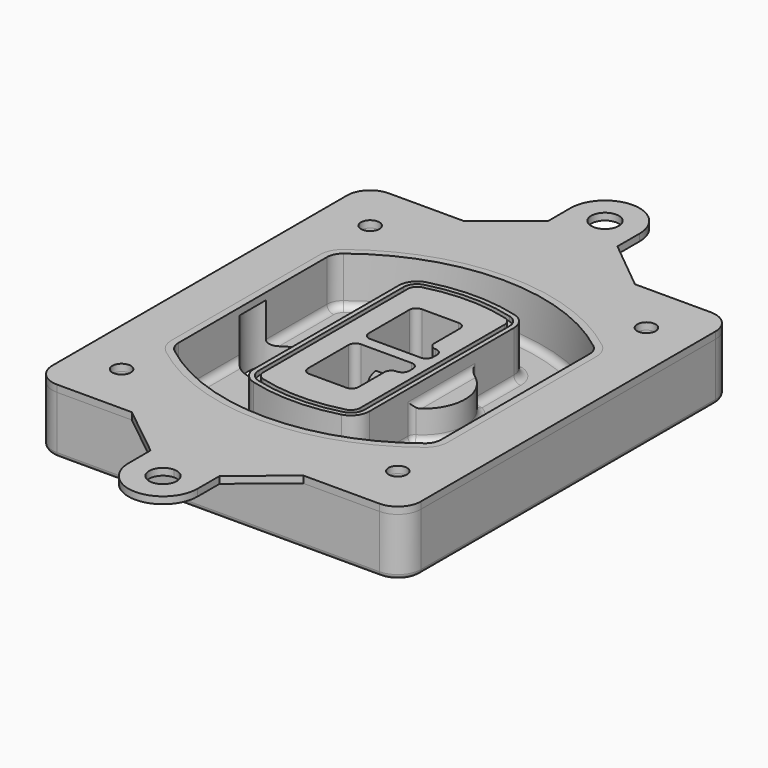
from build123d import *

# Parameters (mm, degrees)
F0_R      = 4
F1_DEPTH  = 25
F2_DEPTH  = 3
F3_DEPTH  = 18
F5_DEPTH  = 21
F6_DEPTH  = 2
F8_DEPTH  = 20
F9_DEPTH  = 16
F10_DEPTH = 25
F7_R      = 6
F7_R_2    = 4
F11_DEPTH = 6
F13_DEPTH = 9
F14_R     = 3
F15_R     = 2
F16_R     = 4
F17_DEPTH = 3
F18_DEPTH = 3
F19_DEPTH = 3


# Not quite as in the source:
# - a feature names something its author has since deleted; it is built from what else it names


with BuildPart() as f1:
    # F0 (on Top) → F1 (new body)
    with BuildSketch(Plane.XY):
        with BuildLine():
            ThreePointArc((-80, -80), (-77.0710678119, -87.0710678119), (-70, -90))
            Line((-70, -90), (70, -90))
            ThreePointArc((70, -90), (77.0710678119, -87.0710678119), (80, -80))
            Line((80, -80), (80, 80))
            ThreePointArc((80, 80), (77.0710678119, 87.0710678119), (70, 90))
            Line((70, 90), (-70, 90))
            ThreePointArc((-70, 90), (-77.0710678119, 87.0710678119), (-80, 80))
            Line((-80, 80), (-80, -80))
        make_face()
        with Locations((-60, -67.5)):
            Circle(F0_R, mode=Mode.SUBTRACT)
        with Locations((60, -67.5)):
            Circle(F0_R, mode=Mode.SUBTRACT)
        with Locations((-60, 67.5)):
            Circle(F0_R, mode=Mode.SUBTRACT)
        with BuildLine():
            ThreePointArc((-64, 40.2934422872), (-62.5820384798, 46.4328484224), (-58.6153846154, 51.3286200352))
            ThreePointArc((-58.6153846154, 51.3286200352), (0, 71.5), (58.6153846154, 51.3286200352))
            ThreePointArc((58.6153846154, 51.3286200352), (62.5820384798, 46.4328484224), (64, 40.2934422872))
            Line((64, 40.2934422872), (64, -40.2934422872))
            ThreePointArc((64, -40.2934422872), (62.5820384798, -46.4328484224), (58.6153846154, -51.3286200352))
            ThreePointArc((58.6153846154, -51.3286200352), (0, -71.5), (-58.6153846154, -51.3286200352))
            ThreePointArc((-58.6153846154, -51.3286200352), (-62.5820384798, -46.4328484224), (-64, -40.2934422872))
            Line((-64, -40.2934422872), (-64, 40.2934422872))
        make_face(mode=Mode.SUBTRACT)
        with Locations((60, 67.5)):
            Circle(F0_R, mode=Mode.SUBTRACT)
        with BuildLine():
            ThreePointArc((58.6153846154, 51.3286200352), (0, 71.5), (-58.6153846154, 51.3286200352))
            ThreePointArc((-58.6153846154, 51.3286200352), (-62.5820384798, 46.4328484224), (-64, 40.2934422872))
            Line((-64, 40.2934422872), (-64, -40.2934422872))
            ThreePointArc((-64, -40.2934422872), (-62.5820384798, -46.4328484224), (-58.6153846154, -51.3286200352))
            ThreePointArc((-58.6153846154, -51.3286200352), (0, -71.5), (58.6153846154, -51.3286200352))
            ThreePointArc((58.6153846154, -51.3286200352), (62.5820384798, -46.4328484224), (64, -40.2934422872))
            Line((64, -40.2934422872), (64, 40.2934422872))
            ThreePointArc((64, 40.2934422872), (62.5820384798, 46.4328484224), (58.6153846154, 51.3286200352))
        make_face()
        with BuildLine():
            Line((-60, -40.2934422872), (-60, 40.2934422872))
            ThreePointArc((-60, 40.2934422872), (-58.9871703427, 44.6787323838), (-56.1538461538, 48.1757121072))
            ThreePointArc((-56.1538461538, 48.1757121072), (0, 67.5), (56.1538461538, 48.1757121072))
            ThreePointArc((56.1538461538, 48.1757121072), (58.9871703427, 44.6787323838), (60, 40.2934422872))
            Line((60, 40.2934422872), (60, -40.2934422872))
            ThreePointArc((60, -40.2934422872), (58.9871703427, -44.6787323838), (56.1538461538, -48.1757121072))
            ThreePointArc((56.1538461538, -48.1757121072), (0, -67.5), (-56.1538461538, -48.1757121072))
            ThreePointArc((-56.1538461538, -48.1757121072), (-58.9871703427, -44.6787323838), (-60, -40.2934422872))
        make_face(mode=Mode.SUBTRACT)
        with BuildLine():
            ThreePointArc((-56.1538461538, 48.1757121072), (-58.9871703427, 44.6787323838), (-60, 40.2934422872))
            Line((-60, 40.2934422872), (-60, -40.2934422872))
            ThreePointArc((-60, -40.2934422872), (-58.9871703427, -44.6787323838), (-56.1538461538, -48.1757121072))
            ThreePointArc((-56.1538461538, -48.1757121072), (0, -67.5), (56.1538461538, -48.1757121072))
            ThreePointArc((56.1538461538, -48.1757121072), (58.9871703427, -44.6787323838), (60, -40.2934422872))
            Line((60, -40.2934422872), (60, 40.2934422872))
            ThreePointArc((60, 40.2934422872), (58.9871703427, 44.6787323838), (56.1538461538, 48.1757121072))
            ThreePointArc((56.1538461538, 48.1757121072), (0, 67.5), (-56.1538461538, 48.1757121072))
        make_face()
        with BuildLine():
            ThreePointArc((54.3076923077, 45.8110311612), (56.2910192399, 43.3631453548), (57, 40.2934422872))
            Line((57, 40.2934422872), (57, -40.2934422872))
            ThreePointArc((57, -40.2934422872), (56.2910192399, -43.3631453548), (54.3076923077, -45.8110311612))
            ThreePointArc((54.3076923077, -45.8110311612), (0, -64.5), (-54.3076923077, -45.8110311612))
            ThreePointArc((-54.3076923077, -45.8110311612), (-56.2910192399, -43.3631453548), (-57, -40.2934422872))
            Line((-57, -40.2934422872), (-57, 40.2934422872))
            ThreePointArc((-57, 40.2934422872), (-56.2910192399, 43.3631453548), (-54.3076923077, 45.8110311612))
            ThreePointArc((-54.3076923077, 45.8110311612), (0, 64.5), (54.3076923077, 45.8110311612))
        make_face(mode=Mode.SUBTRACT)
        with BuildLine():
            Line((57, -40.2934422872), (57, 40.2934422872))
            ThreePointArc((57, 40.2934422872), (56.2910192399, 43.3631453548), (54.3076923077, 45.8110311612))
            ThreePointArc((54.3076923077, 45.8110311612), (0, 64.5), (-54.3076923077, 45.8110311612))
            ThreePointArc((-54.3076923077, 45.8110311612), (-56.2910192399, 43.3631453548), (-57, 40.2934422872))
            Line((-57, 40.2934422872), (-57, -40.2934422872))
            ThreePointArc((-57, -40.2934422872), (-56.2910192399, -43.3631453548), (-54.3076923077, -45.8110311612))
            ThreePointArc((-54.3076923077, -45.8110311612), (0, -64.5), (54.3076923077, -45.8110311612))
            ThreePointArc((54.3076923077, -45.8110311612), (56.2910192399, -43.3631453548), (57, -40.2934422872))
        make_face()
    extrude(amount=-F1_DEPTH)

    # F0 (on Top) → F2 (join)
    with BuildSketch(Plane.XY):
        with BuildLine():
            ThreePointArc((-56.1538461538, 48.1757121072), (-58.9871703427, 44.6787323838), (-60, 40.2934422872))
            Line((-60, 40.2934422872), (-60, -40.2934422872))
            ThreePointArc((-60, -40.2934422872), (-58.9871703427, -44.6787323838), (-56.1538461538, -48.1757121072))
            ThreePointArc((-56.1538461538, -48.1757121072), (0, -67.5), (56.1538461538, -48.1757121072))
            ThreePointArc((56.1538461538, -48.1757121072), (58.9871703427, -44.6787323838), (60, -40.2934422872))
            Line((60, -40.2934422872), (60, 40.2934422872))
            ThreePointArc((60, 40.2934422872), (58.9871703427, 44.6787323838), (56.1538461538, 48.1757121072))
            ThreePointArc((56.1538461538, 48.1757121072), (0, 67.5), (-56.1538461538, 48.1757121072))
        make_face()
        with BuildLine():
            ThreePointArc((54.3076923077, 45.8110311612), (56.2910192399, 43.3631453548), (57, 40.2934422872))
            Line((57, 40.2934422872), (57, -40.2934422872))
            ThreePointArc((57, -40.2934422872), (56.2910192399, -43.3631453548), (54.3076923077, -45.8110311612))
            ThreePointArc((54.3076923077, -45.8110311612), (0, -64.5), (-54.3076923077, -45.8110311612))
            ThreePointArc((-54.3076923077, -45.8110311612), (-56.2910192399, -43.3631453548), (-57, -40.2934422872))
            Line((-57, -40.2934422872), (-57, 40.2934422872))
            ThreePointArc((-57, 40.2934422872), (-56.2910192399, 43.3631453548), (-54.3076923077, 45.8110311612))
            ThreePointArc((-54.3076923077, 45.8110311612), (0, 64.5), (54.3076923077, 45.8110311612))
        make_face(mode=Mode.SUBTRACT)
    extrude(amount=F2_DEPTH)

    # F0 (on Top) → F3 (cut)
    with BuildSketch(Plane.XY):
        with BuildLine():
            Line((57, -40.2934422872), (57, 40.2934422872))
            ThreePointArc((57, 40.2934422872), (56.2910192399, 43.3631453548), (54.3076923077, 45.8110311612))
            ThreePointArc((54.3076923077, 45.8110311612), (0, 64.5), (-54.3076923077, 45.8110311612))
            ThreePointArc((-54.3076923077, 45.8110311612), (-56.2910192399, 43.3631453548), (-57, 40.2934422872))
            Line((-57, 40.2934422872), (-57, -40.2934422872))
            ThreePointArc((-57, -40.2934422872), (-56.2910192399, -43.3631453548), (-54.3076923077, -45.8110311612))
            ThreePointArc((-54.3076923077, -45.8110311612), (0, -64.5), (54.3076923077, -45.8110311612))
            ThreePointArc((54.3076923077, -45.8110311612), (56.2910192399, -43.3631453548), (57, -40.2934422872))
        make_face()
    extrude(amount=-F3_DEPTH, mode=Mode.SUBTRACT)

    # F4 (on face) → F5 (join, through all)
    with BuildSketch(Plane.XY.offset(3)):
        with BuildLine():
            ThreePointArc((-25, -39.2465276821), (-23.3511545998, -44.1109737193), (-19.0842911877, -46.9702398883))
            ThreePointArc((-19.0842911877, -46.9702398883), (0, -49.5), (19.0842911877, -46.9702398883))
            ThreePointArc((19.0842911877, -46.9702398883), (23.3511545998, -44.1109737193), (25, -39.2465276821))
            Line((25, -39.2465276821), (25, 39.2465276821))
            ThreePointArc((25, 39.2465276821), (23.3511545998, 44.1109737193), (19.0842911877, 46.9702398883))
            ThreePointArc((19.0842911877, 46.9702398883), (0, 49.5), (-19.0842911877, 46.9702398883))
            ThreePointArc((-19.0842911877, 46.9702398883), (-23.3511545998, 44.1109737193), (-25, 39.2465276821))
            Line((-25, 39.2465276821), (-25, -39.2465276821))
        make_face()
        with BuildLine():
            ThreePointArc((18.5632183908, 45.0393118368), (21.7633659499, 42.89486221), (23, 39.2465276821))
            Line((23, 39.2465276821), (23, -39.2465276821))
            ThreePointArc((23, -39.2465276821), (21.7633659499, -42.89486221), (18.5632183908, -45.0393118368))
            ThreePointArc((18.5632183908, -45.0393118368), (0, -47.5), (-18.5632183908, -45.0393118368))
            ThreePointArc((-18.5632183908, -45.0393118368), (-21.7633659499, -42.89486221), (-23, -39.2465276821))
            Line((-23, -39.2465276821), (-23, 39.2465276821))
            ThreePointArc((-23, 39.2465276821), (-21.7633659499, 42.89486221), (-18.5632183908, 45.0393118368))
            ThreePointArc((-18.5632183908, 45.0393118368), (0, 47.5), (18.5632183908, 45.0393118368))
        make_face(mode=Mode.SUBTRACT)
        with BuildLine():
            Line((23, -39.2465276821), (23, 39.2465276821))
            ThreePointArc((23, 39.2465276821), (21.7633659499, 42.89486221), (18.5632183908, 45.0393118368))
            ThreePointArc((18.5632183908, 45.0393118368), (0, 47.5), (-18.5632183908, 45.0393118368))
            ThreePointArc((-18.5632183908, 45.0393118368), (-21.7633659499, 42.89486221), (-23, 39.2465276821))
            Line((-23, 39.2465276821), (-23, -39.2465276821))
            ThreePointArc((-23, -39.2465276821), (-21.7633659499, -42.89486221), (-18.5632183908, -45.0393118368))
            ThreePointArc((-18.5632183908, -45.0393118368), (0, -47.5), (18.5632183908, -45.0393118368))
            ThreePointArc((18.5632183908, -45.0393118368), (21.7633659499, -42.89486221), (23, -39.2465276821))
        make_face()
        with BuildLine():
            ThreePointArc((18.0421455939, 43.1083837852), (20.1755772999, 41.6787507007), (21, 39.2465276821))
            Line((21, 39.2465276821), (21, -39.2465276821))
            ThreePointArc((21, -39.2465276821), (20.1755772999, -41.6787507007), (18.0421455939, -43.1083837852))
            ThreePointArc((18.0421455939, -43.1083837852), (0, -45.5), (-18.0421455939, -43.1083837852))
            ThreePointArc((-18.0421455939, -43.1083837852), (-20.1755772999, -41.6787507007), (-21, -39.2465276821))
            Line((-21, -39.2465276821), (-21, 39.2465276821))
            ThreePointArc((-21, 39.2465276821), (-20.1755772999, 41.6787507007), (-18.0421455939, 43.1083837852))
            ThreePointArc((-18.0421455939, 43.1083837852), (0, 45.5), (18.0421455939, 43.1083837852))
        make_face(mode=Mode.SUBTRACT)
        with BuildLine():
            Line((21, -39.2465276821), (21, 39.2465276821))
            ThreePointArc((21, 39.2465276821), (20.1755772999, 41.6787507007), (18.0421455939, 43.1083837852))
            ThreePointArc((18.0421455939, 43.1083837852), (0, 45.5), (-18.0421455939, 43.1083837852))
            ThreePointArc((-18.0421455939, 43.1083837852), (-20.1755772999, 41.6787507007), (-21, 39.2465276821))
            Line((-21, 39.2465276821), (-21, -39.2465276821))
            ThreePointArc((-21, -39.2465276821), (-20.1755772999, -41.6787507007), (-18.0421455939, -43.1083837852))
            ThreePointArc((-18.0421455939, -43.1083837852), (0, -45.5), (18.0421455939, -43.1083837852))
            ThreePointArc((18.0421455939, -43.1083837852), (20.1755772999, -41.6787507007), (21, -39.2465276821))
        make_face()
        with BuildLine():
            Line((-8, -2.5), (14, -2.5))
            ThreePointArc((14, -2.5), (16.1213203436, -3.3786796564), (17, -5.5))
            Line((17, -5.5), (17, -7.5))
            ThreePointArc((17, -7.5), (16.1213203436, -9.6213203436), (14, -10.5))
            ThreePointArc((14, -10.5), (11.8786796564, -11.3786796564), (11, -13.5))
            Line((11, -13.5), (11, -27.5))
            ThreePointArc((11, -27.5), (10.1213203436, -29.6213203436), (8, -30.5))
            Line((8, -30.5), (-8, -30.5))
            ThreePointArc((-8, -30.5), (-10.1213203436, -29.6213203436), (-11, -27.5))
            Line((-11, -27.5), (-11, -5.5))
            ThreePointArc((-11, -5.5), (-10.1213203436, -3.3786796564), (-8, -2.5))
        make_face(mode=Mode.SUBTRACT)
        with BuildLine():
            ThreePointArc((-8, 2.5), (-10.1213203436, 3.3786796564), (-11, 5.5))
            Line((-11, 5.5), (-11, 27.5))
            ThreePointArc((-11, 27.5), (-10.1213203436, 29.6213203436), (-8, 30.5))
            Line((-8, 30.5), (8, 30.5))
            ThreePointArc((8, 30.5), (10.1213203436, 29.6213203436), (11, 27.5))
            Line((11, 27.5), (11, 13.5))
            ThreePointArc((11, 13.5), (11.8786796564, 11.3786796564), (14, 10.5))
            ThreePointArc((14, 10.5), (16.1213203436, 9.6213203436), (17, 7.5))
            Line((17, 7.5), (17, 5.5))
            ThreePointArc((17, 5.5), (16.1213203436, 3.3786796564), (14, 2.5))
            Line((14, 2.5), (-8, 2.5))
        make_face(mode=Mode.SUBTRACT)
    extrude(amount=-F5_DEPTH)

    # F4 (on face) → F6 (cut)
    with BuildSketch(Plane.XY.offset(3)):
        with BuildLine():
            Line((23, -39.2465276821), (23, 39.2465276821))
            ThreePointArc((23, 39.2465276821), (21.7633659499, 42.89486221), (18.5632183908, 45.0393118368))
            ThreePointArc((18.5632183908, 45.0393118368), (0, 47.5), (-18.5632183908, 45.0393118368))
            ThreePointArc((-18.5632183908, 45.0393118368), (-21.7633659499, 42.89486221), (-23, 39.2465276821))
            Line((-23, 39.2465276821), (-23, -39.2465276821))
            ThreePointArc((-23, -39.2465276821), (-21.7633659499, -42.89486221), (-18.5632183908, -45.0393118368))
            ThreePointArc((-18.5632183908, -45.0393118368), (0, -47.5), (18.5632183908, -45.0393118368))
            ThreePointArc((18.5632183908, -45.0393118368), (21.7633659499, -42.89486221), (23, -39.2465276821))
        make_face()
        with BuildLine():
            ThreePointArc((18.0421455939, 43.1083837852), (20.1755772999, 41.6787507007), (21, 39.2465276821))
            Line((21, 39.2465276821), (21, -39.2465276821))
            ThreePointArc((21, -39.2465276821), (20.1755772999, -41.6787507007), (18.0421455939, -43.1083837852))
            ThreePointArc((18.0421455939, -43.1083837852), (0, -45.5), (-18.0421455939, -43.1083837852))
            ThreePointArc((-18.0421455939, -43.1083837852), (-20.1755772999, -41.6787507007), (-21, -39.2465276821))
            Line((-21, -39.2465276821), (-21, 39.2465276821))
            ThreePointArc((-21, 39.2465276821), (-20.1755772999, 41.6787507007), (-18.0421455939, 43.1083837852))
            ThreePointArc((-18.0421455939, 43.1083837852), (0, 45.5), (18.0421455939, 43.1083837852))
        make_face(mode=Mode.SUBTRACT)
    extrude(amount=-F6_DEPTH, mode=Mode.SUBTRACT)

    # F7 (on face) → F8 (join)
    with BuildSketch(Plane(origin=(0, 0, -25), x_dir=(1, 0, 0), z_dir=(0, 0, -1))):
        with BuildLine():
            ThreePointArc((3.28842436, 0), (16.7567035675, 13.4682792075), (30.224982775, 0))
            Line((30.224982775, 0), (35.224982775, 0))
            ThreePointArc((35.224982775, 0), (16.7567035675, 18.4682792075), (-1.71157564, 0))
            Line((-1.71157564, 0), (3.28842436, 0))
        make_face()
        with BuildLine():
            Line((3.28842436, 0), (30.224982775, 0))
            ThreePointArc((30.224982775, 0), (16.7567035675, 13.4682792075), (3.28842436, 0))
        make_face()
        with BuildLine():
            ThreePointArc((3.28842436, 0), (16.7567035675, -13.4682792075), (30.224982775, 0))
            Line((30.224982775, 0), (3.28842436, 0))
        make_face()
        with BuildLine():
            Line((35.224982775, 0), (30.224982775, 0))
            ThreePointArc((30.224982775, 0), (16.7567035675, -13.4682792075), (3.28842436, 0))
            Line((3.28842436, 0), (-1.71157564, 0))
            ThreePointArc((-1.71157564, 0), (16.7567035675, -18.4682792075), (35.224982775, 0))
        make_face()
    extrude(amount=-F8_DEPTH)

    # F7 (on face) → F9 (cut)
    with BuildSketch(Plane(origin=(0, 0, -25), x_dir=(1, 0, 0), z_dir=(0, 0, -1))):
        with BuildLine():
            Line((3.28842436, 0), (30.224982775, 0))
            ThreePointArc((30.224982775, 0), (16.7567035675, 13.4682792075), (3.28842436, 0))
        make_face()
        with BuildLine():
            ThreePointArc((3.28842436, 0), (16.7567035675, -13.4682792075), (30.224982775, 0))
            Line((30.224982775, 0), (3.28842436, 0))
        make_face()
    extrude(amount=-F9_DEPTH, mode=Mode.SUBTRACT)

    # F7 (on face) → F10 (cut)
    with BuildSketch(Plane(origin=(0, 0, -25), x_dir=(1, 0, 0), z_dir=(0, 0, -1))):
        with BuildLine():
            Line((-59.0318229325, 0), (-32.0952645175, 0))
            ThreePointArc((-32.0952645175, 0), (-45.563543725, 13.4682792075), (-59.0318229325, 0))
        make_face()
        with BuildLine():
            ThreePointArc((-59.0318229325, 0), (-45.563543725, -13.4682792075), (-32.0952645175, 0))
            Line((-32.0952645175, 0), (-59.0318229325, 0))
        make_face()
    extrude(amount=-F10_DEPTH, mode=Mode.SUBTRACT)

    # F7 (on face) → F11 (cut)
    with BuildSketch(Plane(origin=(0, 0, -25), x_dir=(1, 0, 0), z_dir=(0, 0, -1))):
        with Locations((60, -67.5)):
            Circle(F7_R)
        with Locations((60, -67.5)):
            Circle(F7_R_2, mode=Mode.SUBTRACT)
        with Locations((-60, -67.5)):
            Circle(F7_R)
        with Locations((-60, -67.5)):
            Circle(F7_R_2, mode=Mode.SUBTRACT)
        with Locations((-60, 67.5)):
            Circle(F7_R)
        with Locations((-60, 67.5)):
            Circle(F7_R_2, mode=Mode.SUBTRACT)
        with Locations((60, 67.5)):
            Circle(F7_R)
        with Locations((60, 67.5)):
            Circle(F7_R_2, mode=Mode.SUBTRACT)
    extrude(amount=-F11_DEPTH, mode=Mode.SUBTRACT)

    # F12 (on face) → F13 (cut, through all)
    with BuildSketch(Plane(origin=(0, 0, -9), x_dir=(1, 0, 0), z_dir=(0, 0, -1))):
        with BuildLine():
            Line((11, 13.5), (11, 17.5481537753))
            ThreePointArc((11, 17.5481537753), (2.5696536419, 11.8239143813), (-1.5415842455, 2.5))
            Line((-1.5415842455, 2.5), (3.5224848595, 2.5))
            ThreePointArc((3.5224848595, 2.5), (6.1857188154, 8.3455872281), (11.2536447004, 12.2927168648))
            ThreePointArc((11.2536447004, 12.2927168648), (11.0640958889, 12.8831798879), (11, 13.5))
        make_face()
        with BuildLine():
            ThreePointArc((11.2536447004, -12.2927168648), (6.1857188154, -8.3455872281), (3.5224848595, -2.5))
            Line((3.5224848595, -2.5), (-1.5415842455, -2.5))
            ThreePointArc((-1.5415842455, -2.5), (2.5696536419, -11.8239143813), (11, -17.5481537753))
            Line((11, -17.5481537753), (11, -13.5))
            ThreePointArc((11, -13.5), (11.0640958889, -12.8831798879), (11.2536447004, -12.2927168648))
        make_face()
        with BuildLine():
            ThreePointArc((11.2536447004, 12.2927168648), (6.1857188154, 8.3455872281), (3.5224848595, 2.5))
            Line((3.5224848595, 2.5), (14, 2.5))
            ThreePointArc((14, 2.5), (16.1213203436, 3.3786796564), (17, 5.5))
            Line((17, 5.5), (17, 7.5))
            ThreePointArc((17, 7.5), (16.1213203436, 9.6213203436), (14, 10.5))
            ThreePointArc((14, 10.5), (12.3601599782, 10.9878446101), (11.2536447004, 12.2927168648))
        make_face()
        with BuildLine():
            Line((14, -2.5), (3.5224848595, -2.5))
            ThreePointArc((3.5224848595, -2.5), (6.1857188154, -8.3455872281), (11.2536447004, -12.2927168648))
            ThreePointArc((11.2536447004, -12.2927168648), (12.3601599782, -10.9878446101), (14, -10.5))
            ThreePointArc((14, -10.5), (16.1213203436, -9.6213203436), (17, -7.5))
            Line((17, -7.5), (17, -5.5))
            ThreePointArc((17, -5.5), (16.1213203436, -3.3786796564), (14, -2.5))
        make_face()
    extrude(amount=F13_DEPTH, mode=Mode.SUBTRACT)

    # F14
    f14_edges = [f1.edges().sort_by_distance(p)[0] for p in [
        (-57, -23.703476, -18),
        (-57, 23.703476, -18),
        (25, 0, -5),
        (25, 16.526506, -11.5),
        (25, -16.526506, -11.5),
        (25, -27.886517, -18),
        (35.224983, 0, -18),
    ]]
    fillet(f14_edges, radius=F14_R)

    # F15
    f15_edges = [f1.edges().sort_by_distance(p)[0] for p in [
        (0, -90, -25),
    ]]
    fillet(f15_edges, radius=F15_R)


with BuildPart() as f17:
    # F16 (on face) → F17 (new body, through all)
    with BuildSketch(Plane.XY):
        with BuildLine():
            Line((-80, 80), (-80, -80))
            ThreePointArc((-80, -80), (-77.0710678119, -87.0710678119), (-70, -90))
            Line((-70, -90), (-37.5495068729, -90))
            Line((-37.5495068729, -90), (0, -90))
            Line((0, -90), (37.0184704661, -90))
            Line((37.0184704661, -90), (70, -90))
            ThreePointArc((70, -90), (77.0710678119, -87.0710678119), (80, -80))
            Line((80, -80), (80, 80))
            ThreePointArc((80, 80), (77.0710678119, 87.0710678119), (70, 90))
            Line((70, 90), (37.0184704661, 90))
            Line((37.0184704661, 90), (0, 90))
            Line((0, 90), (-37.5495068729, 90))
            Line((-37.5495068729, 90), (-70, 90))
            ThreePointArc((-70, 90), (-77.0710678119, 87.0710678119), (-80, 80))
        make_face()
        with Locations((-60, -67.5)):
            Circle(F16_R, mode=Mode.SUBTRACT)
        with Locations((60, -67.5)):
            Circle(F16_R, mode=Mode.SUBTRACT)
        with Locations((-60, 67.5)):
            Circle(F16_R, mode=Mode.SUBTRACT)
        with BuildLine():
            ThreePointArc((-56.1538461538, 48.1757121072), (0, 67.5), (56.1538461538, 48.1757121072))
            ThreePointArc((56.1538461538, 48.1757121072), (58.9871703427, 44.6787323838), (60, 40.2934422872))
            Line((60, 40.2934422872), (60, -40.2934422872))
            ThreePointArc((60, -40.2934422872), (58.9871703427, -44.6787323838), (56.1538461538, -48.1757121072))
            ThreePointArc((56.1538461538, -48.1757121072), (0, -67.5), (-56.1538461538, -48.1757121072))
            ThreePointArc((-56.1538461538, -48.1757121072), (-58.9871703427, -44.6787323838), (-60, -40.2934422872))
            Line((-60, -40.2934422872), (-60, 40.2934422872))
            ThreePointArc((-60, 40.2934422872), (-58.9871703427, 44.6787323838), (-56.1538461538, 48.1757121072))
        make_face(mode=Mode.SUBTRACT)
        with Locations((60, 67.5)):
            Circle(F16_R, mode=Mode.SUBTRACT)
        with BuildLine():
            Line((-15, 108), (-37.5495068729, 90))
            Line((-37.5495068729, 90), (0, 90))
            Line((0, 90), (37.0184704661, 90))
            Line((37.0184704661, 90), (15, 108))
            Line((15, 108), (15, 120))
            ThreePointArc((15, 120), (0, 135), (-15, 120))
            Line((-15, 120), (-15, 108))
        make_face()
        with BuildLine():
            ThreePointArc((6, 120), (4.2426406871, 115.7573593129), (0, 114))
            ThreePointArc((0, 114), (-4.2426406871, 124.2426406871), (6, 120))
        make_face(mode=Mode.SUBTRACT)
    extrude(amount=F17_DEPTH)


with BuildPart() as f18:
    # F16 (on face) → F18 (new body, through all)
    with BuildSketch(Plane.XY):
        with BuildLine():
            Line((-80, 80), (-80, -80))
            ThreePointArc((-80, -80), (-77.0710678119, -87.0710678119), (-70, -90))
            Line((-70, -90), (-37.5495068729, -90))
            Line((-37.5495068729, -90), (0, -90))
            Line((0, -90), (37.0184704661, -90))
            Line((37.0184704661, -90), (70, -90))
            ThreePointArc((70, -90), (77.0710678119, -87.0710678119), (80, -80))
            Line((80, -80), (80, 80))
            ThreePointArc((80, 80), (77.0710678119, 87.0710678119), (70, 90))
            Line((70, 90), (37.0184704661, 90))
            Line((37.0184704661, 90), (0, 90))
            Line((0, 90), (-37.5495068729, 90))
            Line((-37.5495068729, 90), (-70, 90))
            ThreePointArc((-70, 90), (-77.0710678119, 87.0710678119), (-80, 80))
        make_face()
        with Locations((-60, -67.5)):
            Circle(F16_R, mode=Mode.SUBTRACT)
        with Locations((60, -67.5)):
            Circle(F16_R, mode=Mode.SUBTRACT)
        with Locations((-60, 67.5)):
            Circle(F16_R, mode=Mode.SUBTRACT)
        with BuildLine():
            ThreePointArc((-56.1538461538, 48.1757121072), (0, 67.5), (56.1538461538, 48.1757121072))
            ThreePointArc((56.1538461538, 48.1757121072), (58.9871703427, 44.6787323838), (60, 40.2934422872))
            Line((60, 40.2934422872), (60, -40.2934422872))
            ThreePointArc((60, -40.2934422872), (58.9871703427, -44.6787323838), (56.1538461538, -48.1757121072))
            ThreePointArc((56.1538461538, -48.1757121072), (0, -67.5), (-56.1538461538, -48.1757121072))
            ThreePointArc((-56.1538461538, -48.1757121072), (-58.9871703427, -44.6787323838), (-60, -40.2934422872))
            Line((-60, -40.2934422872), (-60, 40.2934422872))
            ThreePointArc((-60, 40.2934422872), (-58.9871703427, 44.6787323838), (-56.1538461538, 48.1757121072))
        make_face(mode=Mode.SUBTRACT)
        with Locations((60, 67.5)):
            Circle(F16_R, mode=Mode.SUBTRACT)
        with BuildLine():
            Line((0, -90), (-37.5495068729, -90))
            Line((-37.5495068729, -90), (-15, -108))
            Line((-15, -108), (-15, -120))
            ThreePointArc((-15, -120), (0, -135), (15, -120))
            Line((15, -120), (15, -108))
            Line((15, -108), (37.0184704661, -90))
            Line((37.0184704661, -90), (0, -90))
        make_face()
        with BuildLine():
            ThreePointArc((6, -120), (-4.2426406871, -124.2426406871), (0, -114))
            ThreePointArc((0, -114), (4.2426406871, -115.7573593129), (6, -120))
        make_face(mode=Mode.SUBTRACT)
        with BuildLine():
            Line((-15, 108), (-37.5495068729, 90))
            Line((-37.5495068729, 90), (0, 90))
            Line((0, 90), (37.0184704661, 90))
            Line((37.0184704661, 90), (15, 108))
            Line((15, 108), (15, 120))
            ThreePointArc((15, 120), (0, 135), (-15, 120))
            Line((-15, 120), (-15, 108))
        make_face()
        with BuildLine():
            ThreePointArc((6, 120), (4.2426406871, 115.7573593129), (0, 114))
            ThreePointArc((0, 114), (-4.2426406871, 124.2426406871), (6, 120))
        make_face(mode=Mode.SUBTRACT)
    extrude(amount=F18_DEPTH)


with BuildPart() as f19:
    # F16 (on face) → F19 (new body, through all)
    with BuildSketch(Plane.XY):
        with BuildLine():
            Line((-15, 108), (-37.5495068729, 90))
            Line((-37.5495068729, 90), (0, 90))
            Line((0, 90), (37.0184704661, 90))
            Line((37.0184704661, 90), (15, 108))
            Line((15, 108), (15, 120))
            ThreePointArc((15, 120), (0, 135), (-15, 120))
            Line((-15, 120), (-15, 108))
        make_face()
        with BuildLine():
            ThreePointArc((6, 120), (4.2426406871, 115.7573593129), (0, 114))
            ThreePointArc((0, 114), (-4.2426406871, 124.2426406871), (6, 120))
        make_face(mode=Mode.SUBTRACT)
        with BuildLine():
            Line((-80, 80), (-80, -80))
            ThreePointArc((-80, -80), (-77.0710678119, -87.0710678119), (-70, -90))
            Line((-70, -90), (-37.5495068729, -90))
            Line((-37.5495068729, -90), (0, -90))
            Line((0, -90), (37.0184704661, -90))
            Line((37.0184704661, -90), (70, -90))
            ThreePointArc((70, -90), (77.0710678119, -87.0710678119), (80, -80))
            Line((80, -80), (80, 80))
            ThreePointArc((80, 80), (77.0710678119, 87.0710678119), (70, 90))
            Line((70, 90), (37.0184704661, 90))
            Line((37.0184704661, 90), (0, 90))
            Line((0, 90), (-37.5495068729, 90))
            Line((-37.5495068729, 90), (-70, 90))
            ThreePointArc((-70, 90), (-77.0710678119, 87.0710678119), (-80, 80))
        make_face()
        with Locations((-60, -67.5)):
            Circle(F16_R, mode=Mode.SUBTRACT)
        with Locations((60, -67.5)):
            Circle(F16_R, mode=Mode.SUBTRACT)
        with Locations((-60, 67.5)):
            Circle(F16_R, mode=Mode.SUBTRACT)
        with BuildLine():
            ThreePointArc((-56.1538461538, 48.1757121072), (0, 67.5), (56.1538461538, 48.1757121072))
            ThreePointArc((56.1538461538, 48.1757121072), (58.9871703427, 44.6787323838), (60, 40.2934422872))
            Line((60, 40.2934422872), (60, -40.2934422872))
            ThreePointArc((60, -40.2934422872), (58.9871703427, -44.6787323838), (56.1538461538, -48.1757121072))
            ThreePointArc((56.1538461538, -48.1757121072), (0, -67.5), (-56.1538461538, -48.1757121072))
            ThreePointArc((-56.1538461538, -48.1757121072), (-58.9871703427, -44.6787323838), (-60, -40.2934422872))
            Line((-60, -40.2934422872), (-60, 40.2934422872))
            ThreePointArc((-60, 40.2934422872), (-58.9871703427, 44.6787323838), (-56.1538461538, 48.1757121072))
        make_face(mode=Mode.SUBTRACT)
        with Locations((60, 67.5)):
            Circle(F16_R, mode=Mode.SUBTRACT)
        with BuildLine():
            Line((0, -90), (-37.5495068729, -90))
            Line((-37.5495068729, -90), (-15, -108))
            Line((-15, -108), (-15, -120))
            ThreePointArc((-15, -120), (0, -135), (15, -120))
            Line((15, -120), (15, -108))
            Line((15, -108), (37.0184704661, -90))
            Line((37.0184704661, -90), (0, -90))
        make_face()
        with BuildLine():
            ThreePointArc((6, -120), (-4.2426406871, -124.2426406871), (0, -114))
            ThreePointArc((0, -114), (4.2426406871, -115.7573593129), (6, -120))
        make_face(mode=Mode.SUBTRACT)
    extrude(amount=F19_DEPTH)


solid = Compound([f1.part, f18.part, f19.part])
